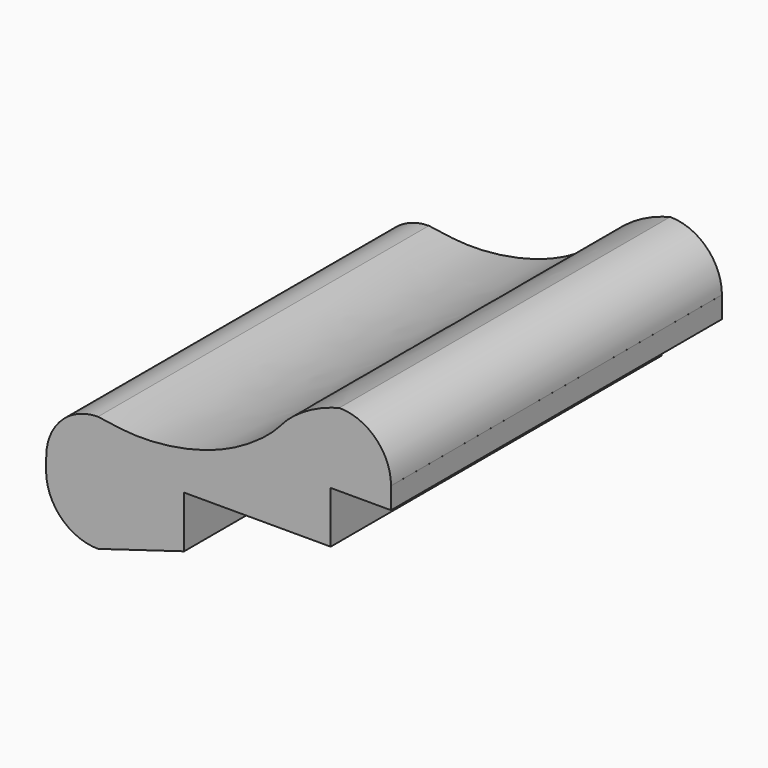
from build123d import *

# Parameters (mm, degrees)
F1_DEPTH = 152.4


# Not quite as in the source:
# - a feature of the source that left no trace in its solid (it failed there, or was rolled back) is left out


with BuildPart() as f1:
    # F0 (on Front) → F1 (new body)
    with BuildSketch(Plane.XZ):
        with BuildLine():
            Line((63.5156407952, 10.3399762884), (63.5156407952, 18.2530842721))
            Line((63.5156407952, 18.2530842721), (63.5201856653, 18.2612892249))
            ThreePointArc((63.5201856653, 18.2612892249), (57.9382188033, 31.7375402421), (44.462159276, 37.3199693859))
            add(Edge.make_bspline(
                [(-44.4622051984, 5.5512220147), (-39.4489640202, 4.7743889629), (-28.8914565164, 3.1384371939), (-9.7165157973, 5.4821340103), (7.2225801678, 11.7489232999), (20.3909952314, 21.2138869863), (25.1500405302, 27.747417878), (33.6683098111, 33.4923986759), (40.5448826371, 36.2228742762), (43.3047932524, 36.9958307759), (44.462159276, 37.3199693859)],
                knots=[0, 0, 0, 0, 0.1447564987, 0.3048462595, 0.4628693182, 0.6074722668, 0.711629737, 0.827910892, 0.927834588, 1, 1, 1, 1], degree=3))
            ThreePointArc((-44.4622051984, 5.5512220147), (-57.9390215503, -0.0226415893), (-63.5199193484, -13.4965465253))
            Line((-63.5199193484, -13.4965465253), (-63.5854476605, -18.2502795355))
            ThreePointArc((-63.5854476605, -18.2502795355), (-57.9464666974, -31.7561163984), (-44.400241226, -37.2973717749))
            Line((-44.400241226, -37.2973717749), (-12.7040622756, -27.7813021094))
            Line((-12.7040622756, -27.7813021094), (-12.7040622756, -8.7301339954))
            Line((-12.7040622756, -8.7301339954), (41.2755347788, -8.7301339954))
            Line((41.2755347788, -8.7301339954), (41.2755347788, 10.3399762884))
            Line((41.2755347788, 10.3399762884), (63.5156407952, 10.3399762884))
        make_face()
    extrude(amount=F1_DEPTH)


solid = f1.part
